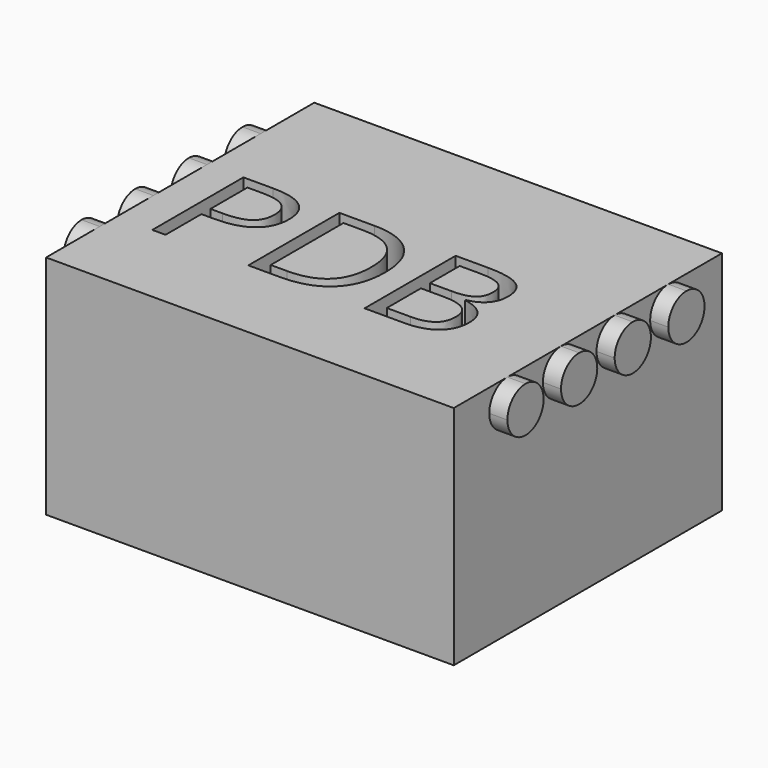
from build123d import *

# Parameters (mm, degrees)
F0_W         = 45
F0_H         = 37
F1_DEPTH     = 25
F3_DEPTH     = 2
F5_DEPTH     = 2
F6_TEXT_SIZE = 17.5989943432
F7_DEPTH     = 25.4


# Not quite as in the source:
# - Text() gives the source's letters only with a copy of the font that has no kerning and outlines rounded to 1/6400 em; it was checked with that copy


with BuildPart() as f1:
    # F0 (on Top) → F1 (new body)
    with BuildSketch(Plane.XY):
        Rectangle(F0_W, F0_H)
    extrude(amount=F1_DEPTH)

    # F6 (on face) → F7 (cut)
    with BuildSketch(Plane.XY.offset(25)):
        with Locations((-20.2873099296, -8.7647953675)):
            Text('PDB', F6_TEXT_SIZE, font='Open Sans', text_align=(TextAlign.LEFT, TextAlign.BOTTOM))
    extrude(amount=-F7_DEPTH, mode=Mode.SUBTRACT)


with BuildPart() as f3:
    # F2 (on face) → F3 (new body)
    with BuildSketch(Plane(origin=(-22.5, 0, 0), x_dir=(0, -1, 0), z_dir=(-1, 0, 0))):
        with BuildLine():
            Line((-11.1, 22.5), (-8.6, 22.5))
            ThreePointArc((-8.6, 22.5), (-9.3322330441, 24.2677669501), (-11.0999999918, 25))
            ThreePointArc((-11.0999999918, 25), (-12.8677669501, 24.2677669559), (-13.6, 22.5))
            Line((-13.6, 22.5), (-11.1, 22.5))
        make_face()
        with BuildLine():
            ThreePointArc((-13.6, 22.5), (-11.1, 20), (-8.6, 22.5))
            Line((-8.6, 22.5), (-11.1, 22.5))
            Line((-11.1, 22.5), (-13.6, 22.5))
        make_face()
    extrude(amount=F3_DEPTH)


with BuildPart() as f3b:
    # F2 (on face) → F3, piece 2 (new body)
    with BuildSketch(Plane(origin=(-22.5, 0, 0), x_dir=(0, -1, 0), z_dir=(-1, 0, 0))):
        with BuildLine():
            Line((-3.7, 22.5), (-6.2, 22.5))
            ThreePointArc((-6.2, 22.5), (-3.7, 20), (-1.2, 22.5))
            Line((-1.2, 22.5), (-3.7, 22.5))
        make_face()
        with BuildLine():
            ThreePointArc((-3.7, 25), (-5.467766953, 24.267766953), (-6.2, 22.5))
            Line((-6.2, 22.5), (-3.7, 22.5))
            Line((-3.7, 22.5), (-1.2, 22.5))
            ThreePointArc((-1.2, 22.5), (-1.932233047, 24.267766953), (-3.7, 25))
        make_face()
    extrude(amount=F3_DEPTH)


with BuildPart() as f3c:
    # F2 (on face) → F3, piece 3 (new body)
    with BuildSketch(Plane(origin=(-22.5, 0, 0), x_dir=(0, -1, 0), z_dir=(-1, 0, 0))):
        with BuildLine():
            ThreePointArc((6.2, 22.5), (5.467766953, 24.267766953), (3.7, 25))
            ThreePointArc((3.7, 25), (1.932233047, 24.267766953), (1.2, 22.5))
            Line((1.2, 22.5), (3.7, 22.5))
            Line((3.7, 22.5), (6.2, 22.5))
        make_face()
        with BuildLine():
            Line((3.7, 22.5), (1.2, 22.5))
            ThreePointArc((1.2, 22.5), (3.7, 20), (6.2, 22.5))
            Line((6.2, 22.5), (3.7, 22.5))
        make_face()
    extrude(amount=F3_DEPTH)


with BuildPart() as f3d:
    # F2 (on face) → F3, piece 4 (new body)
    with BuildSketch(Plane(origin=(-22.5, 0, 0), x_dir=(0, -1, 0), z_dir=(-1, 0, 0))):
        with BuildLine():
            ThreePointArc((13.6, 22.5), (12.867766953, 24.267766953), (11.1, 25))
            ThreePointArc((11.1, 25), (9.332233047, 24.267766953), (8.6, 22.5))
            Line((8.6, 22.5), (11.1, 22.5))
            Line((11.1, 22.5), (13.6, 22.5))
        make_face()
        with BuildLine():
            Line((11.1, 22.5), (8.6, 22.5))
            ThreePointArc((8.6, 22.5), (11.1, 20), (13.6, 22.5))
            Line((13.6, 22.5), (11.1, 22.5))
        make_face()
    extrude(amount=F3_DEPTH)


with BuildPart() as f5:
    # F4 (on face) → F5 (new body)
    with BuildSketch(Plane.YZ.offset(22.5)):
        with BuildLine():
            Line((-11.1, 22.5), (-8.6, 22.5))
            ThreePointArc((-8.6, 22.5), (-9.3322330441, 24.2677669501), (-11.0999999918, 25))
            ThreePointArc((-11.0999999918, 25), (-12.8677669501, 24.2677669559), (-13.6, 22.5))
            Line((-13.6, 22.5), (-11.1, 22.5))
        make_face()
        with BuildLine():
            ThreePointArc((-13.6, 22.5), (-11.1, 20), (-8.6, 22.5))
            Line((-8.6, 22.5), (-11.1, 22.5))
            Line((-11.1, 22.5), (-13.6, 22.5))
        make_face()
    extrude(amount=F5_DEPTH)


with BuildPart() as f5b:
    # F4 (on face) → F5, piece 2 (new body)
    with BuildSketch(Plane.YZ.offset(22.5)):
        with BuildLine():
            ThreePointArc((-3.7, 25), (-5.467766953, 24.267766953), (-6.2, 22.5))
            Line((-6.2, 22.5), (-3.7, 22.5))
            Line((-3.7, 22.5), (-1.2, 22.5))
            ThreePointArc((-1.2, 22.5), (-1.932233047, 24.267766953), (-3.7, 25))
        make_face()
        with BuildLine():
            Line((-3.7, 22.5), (-6.2, 22.5))
            ThreePointArc((-6.2, 22.5), (-3.7, 20), (-1.2, 22.5))
            Line((-1.2, 22.5), (-3.7, 22.5))
        make_face()
    extrude(amount=F5_DEPTH)


with BuildPart() as f5c:
    # F4 (on face) → F5, piece 3 (new body)
    with BuildSketch(Plane.YZ.offset(22.5)):
        with BuildLine():
            ThreePointArc((6.2, 22.5), (5.467766953, 24.267766953), (3.7, 25))
            ThreePointArc((3.7, 25), (1.932233047, 24.267766953), (1.2, 22.5))
            Line((1.2, 22.5), (3.7, 22.5))
            Line((3.7, 22.5), (6.2, 22.5))
        make_face()
        with BuildLine():
            Line((3.7, 22.5), (1.2, 22.5))
            ThreePointArc((1.2, 22.5), (3.7, 20), (6.2, 22.5))
            Line((6.2, 22.5), (3.7, 22.5))
        make_face()
    extrude(amount=F5_DEPTH)


with BuildPart() as f5d:
    # F4 (on face) → F5, piece 4 (new body)
    with BuildSketch(Plane.YZ.offset(22.5)):
        with BuildLine():
            ThreePointArc((13.6, 22.5), (12.867766953, 24.267766953), (11.1, 25))
            ThreePointArc((11.1, 25), (9.332233047, 24.267766953), (8.6, 22.5))
            Line((8.6, 22.5), (11.1, 22.5))
            Line((11.1, 22.5), (13.6, 22.5))
        make_face()
        with BuildLine():
            Line((11.1, 22.5), (8.6, 22.5))
            ThreePointArc((8.6, 22.5), (11.1, 20), (13.6, 22.5))
            Line((13.6, 22.5), (11.1, 22.5))
        make_face()
    extrude(amount=F5_DEPTH)


solid = Compound([f1.part, f3.part, f3b.part, f3c.part, f3d.part, f5.part, f5b.part, f5c.part, f5d.part])
